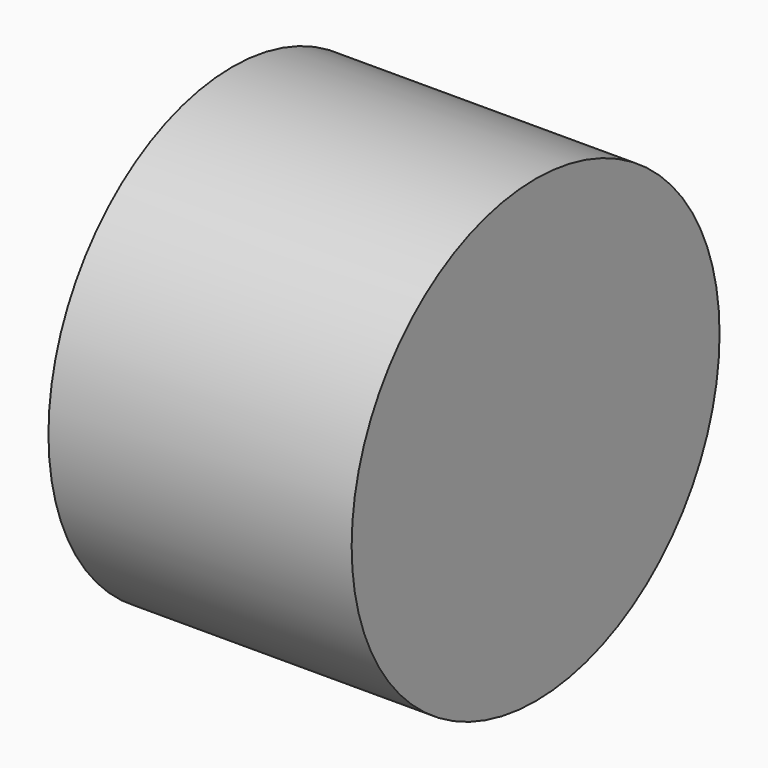
from build123d import *

# Parameters (mm, degrees)
F0_W = 55.0629943609
F0_H = 41.7591929436


# Not quite as in the source:
# - the program builds the solid bodies; features that only make, move or delete a surface that nothing else refers to are left out


with BuildPart() as f2:
    # F0 (on Front) → F2 (revolve)
    with BuildSketch(Plane.XZ):
        with Locations((27.5314971805, 20.8795964718)):
            Rectangle(F0_W, F0_H)
    revolve(axis=Axis((27.5314971805, 0, 0), (-1, 0, 0)))


solid = f2.part
